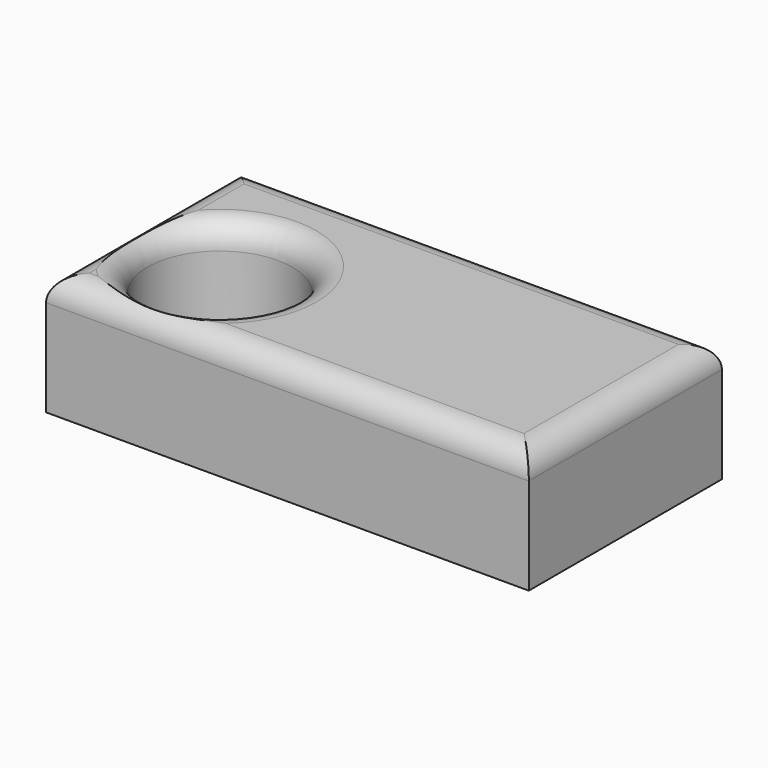
from build123d import *

# Parameters (mm, degrees)
F0_W        = 100
F0_H        = 50
F1_DEPTH    = 25
F2_R        = 15
F3_DEPTH    = 25.001
F4_T1_DEPTH = 75
F4_T3_DEPTH = 125


# Not quite as in the source:
# - a fillet or chamfer that OpenCascade refuses, or shapes differently, is made with other operations: its cross-section is extruded or revolved along the edge and cut away or added


with BuildPart() as f1:
    # F0 (on Top) → F1 (new body)
    with BuildSketch(Plane.XY):
        with Locations((50, 25)):
            Rectangle(F0_W, F0_H)
    extrude(amount=F1_DEPTH)

    # F2 (on face) → F3 (cut, through all)
    with BuildSketch(Plane.XY.offset(25)):
        with Locations((20, 20)):
            Circle(F2_R)
    extrude(amount=-F3_DEPTH, mode=Mode.SUBTRACT)

    # F4: fillet of radius 5 on 5 edges, made by hand

    # F4_s2 → F4_t1 (cut)
    with BuildSketch(Plane.XZ.offset(-62.5)):
        with BuildLine():
            ThreePointArc((0, 20), (1.4644660941, 23.5355339059), (5, 25))
            Line((5, 25), (0, 25))
            Line((0, 25), (0, 20))
        make_face()
        with BuildLine():
            ThreePointArc((95, 25), (98.5355339059, 23.5355339059), (100, 20))
            Line((100, 20), (100, 25))
            Line((100, 25), (95, 25))
        make_face()
    extrude(amount=F4_T1_DEPTH, mode=Mode.SUBTRACT)

    # F4_s4 → F4_t3 (cut)
    with BuildSketch(Plane.YZ.offset(-12.5)):
        with BuildLine():
            ThreePointArc((50, 20), (48.5355339059, 23.5355339059), (45, 25))
            Line((45, 25), (50, 25))
            Line((50, 25), (50, 20))
        make_face()
        with BuildLine():
            ThreePointArc((0, 20), (1.4644660941, 23.5355339059), (5, 25))
            Line((5, 25), (0, 25))
            Line((0, 25), (0, 20))
        make_face()
    extrude(amount=F4_T3_DEPTH, mode=Mode.SUBTRACT)

    # F4_s5 → F4_t6 (revolve, cut)
    with BuildSketch(Plane.XZ.offset(-20)):
        with BuildLine():
            ThreePointArc((40, 25), (36.4644660941, 23.5355339059), (35, 20))
            Line((35, 20), (35, 25))
            Line((35, 25), (40, 25))
        make_face()
    revolve(axis=Axis((20, 20, 25), (0, 0, 1)), mode=Mode.SUBTRACT)


solid = f1.part
